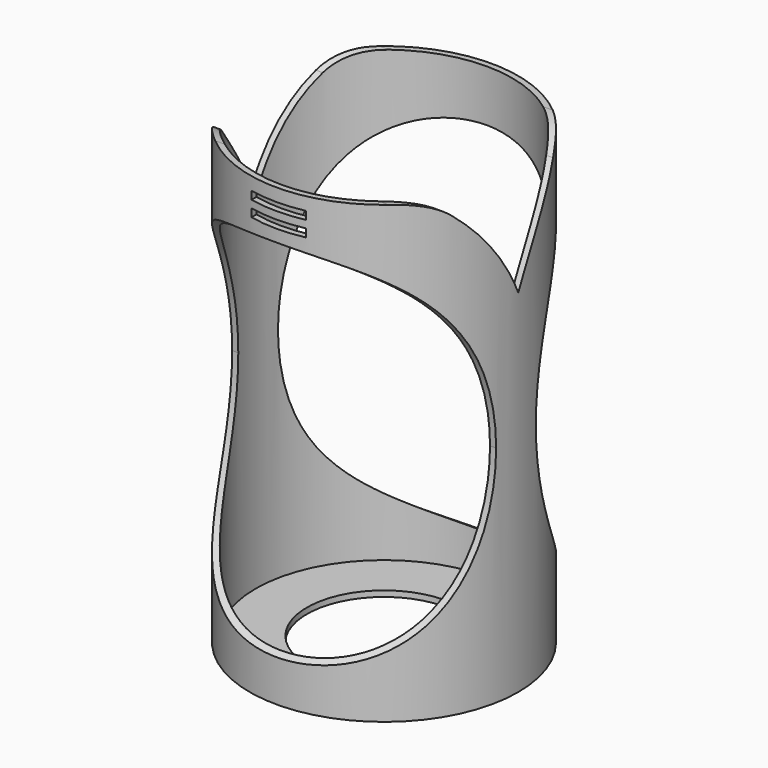
from build123d import *

# Parameters (mm, degrees)
F0_R         = 39.37
F1_DEPTH     = 1.778
F2_R         = 40.3543101783
F3_DEPTH     = 1.778
F4_R         = 23.6510433677
F5_DEPTH     = 25.4
F6_R         = 41.2236595875
F6_R_2       = 39.37
F7_DEPTH     = 139.7
F9_R         = 63.5
F10_DEPTH    = 193.6246595875
F12_W        = 16.764
F12_H        = 2.4538338184
F13_DEPTH    = 101.6
F14_T1_DEPTH = 39.0530419586
F14_T3_DEPTH = 39.0530419586


# Not quite as in the source:
# - a fillet or chamfer that OpenCascade refuses, or shapes differently, is made with other operations: its cross-section is extruded or revolved along the edge and cut away or added


with BuildPart() as f1:
    # F0 (on Top) → F1 (new body)
    with BuildSketch(Plane.XY):
        Circle(F0_R)
    extrude(amount=F1_DEPTH)

    # F2 (on face) → F3 (join)
    with BuildSketch(Plane.XY):
        Circle(F2_R)
    extrude(amount=F3_DEPTH)

    # F4 (on face) → F5 (cut)
    with BuildSketch(Plane.XY):
        Circle(F4_R)
    extrude(amount=F5_DEPTH, mode=Mode.SUBTRACT)

    # F6 (on face) → F7 (join)
    with BuildSketch(Plane.XY):
        Circle(F6_R)
        Circle(F6_R_2, mode=Mode.SUBTRACT)
    extrude(amount=F7_DEPTH)

    # F9 (on offset) → F10 (cut, through all)
    with BuildSketch(Plane.YZ.offset(152.4)):
        with BuildLine():
            ThreePointArc((-25.4, 140.0532810314), (-10.7002122115, 125.5814069058), (0, 107.9455241561))
            Line((0, 107.9455241561), (0, 140.0532810314))
            Line((0, 140.0532810314), (-25.4, 140.0532810314))
        make_face()
        with BuildLine():
            Line((0, 140.0532810314), (0, 107.9455241561))
            ThreePointArc((0, 107.9455241561), (10.7002122115, 125.5814069058), (25.4, 140.0532810314))
            Line((25.4, 140.0532810314), (0, 140.0532810314))
        make_face()
        with BuildLine():
            ThreePointArc((134.62, 68.8011486912), (71.12, 132.3011486912), (7.62, 68.8011486912))
            ThreePointArc((7.62, 68.8011486912), (71.12, 5.3011486912), (134.62, 68.8011486912))
        make_face()
        with Locations((-71.12, 68.8011486912)):
            Circle(F9_R)
    extrude(amount=-F10_DEPTH, mode=Mode.SUBTRACT)

    # F12 (on offset) → F13 (cut)
    with BuildSketch(Plane.XZ.offset(76.2)):
        Polygon((-8.382, 128.5605213805), (0, 128.5605213805), (8.382, 128.5605213805), (8.382, 131.0175483104), (-8.382, 131.0175483104), align=None)
        with Locations((0, 134.5272064209)):
            Rectangle(F12_W, F12_H)
    extrude(amount=-F13_DEPTH, mode=Mode.SUBTRACT)

    # F14: fillet of radius 17.78 on 4 edges, made by hand

    # F14_s2 → F14_t1 (cut)
    with BuildSketch(Plane.YZ.offset(-51.1681473426)):
        with BuildLine():
            ThreePointArc((-31.4518922665, 139.7), (-24.9514267372, 138.4690890354), (-19.3510168091, 134.9467882905))
            ThreePointArc((-19.3510168091, 134.9467882905), (-22.0942714255, 137.3848907871), (-24.9420879587, 139.7))
            Line((-24.9420879587, 139.7), (-31.4518922665, 139.7))
        make_face()
        with BuildLine():
            ThreePointArc((19.3510168091, 134.9467882905), (24.9514267372, 138.4690890354), (31.4518922665, 139.7))
            Line((31.4518922665, 139.7), (24.9420879587, 139.7))
            ThreePointArc((24.9420879587, 139.7), (22.0942714255, 137.3848907871), (19.3510168091, 134.9467882905))
        make_face()
    extrude(amount=F14_T1_DEPTH, mode=Mode.SUBTRACT)

    # F14_s4 → F14_t3 (cut)
    with BuildSketch(Plane.YZ.offset(12.115105384)):
        with BuildLine():
            ThreePointArc((-19.3510168091, 134.9467882905), (-24.9514267372, 138.4690890354), (-31.4518922665, 139.7))
            Line((-31.4518922665, 139.7), (-24.9420879587, 139.7))
            ThreePointArc((-24.9420879587, 139.7), (-22.0942714255, 137.3848907871), (-19.3510168091, 134.9467882905))
        make_face()
        with BuildLine():
            ThreePointArc((31.4518922665, 139.7), (24.9514267372, 138.4690890354), (19.3510168091, 134.9467882905))
            ThreePointArc((19.3510168091, 134.9467882905), (22.0942714255, 137.3848907871), (24.9420879587, 139.7))
            Line((24.9420879587, 139.7), (31.4518922665, 139.7))
        make_face()
    extrude(amount=F14_T3_DEPTH, mode=Mode.SUBTRACT)


solid = f1.part
